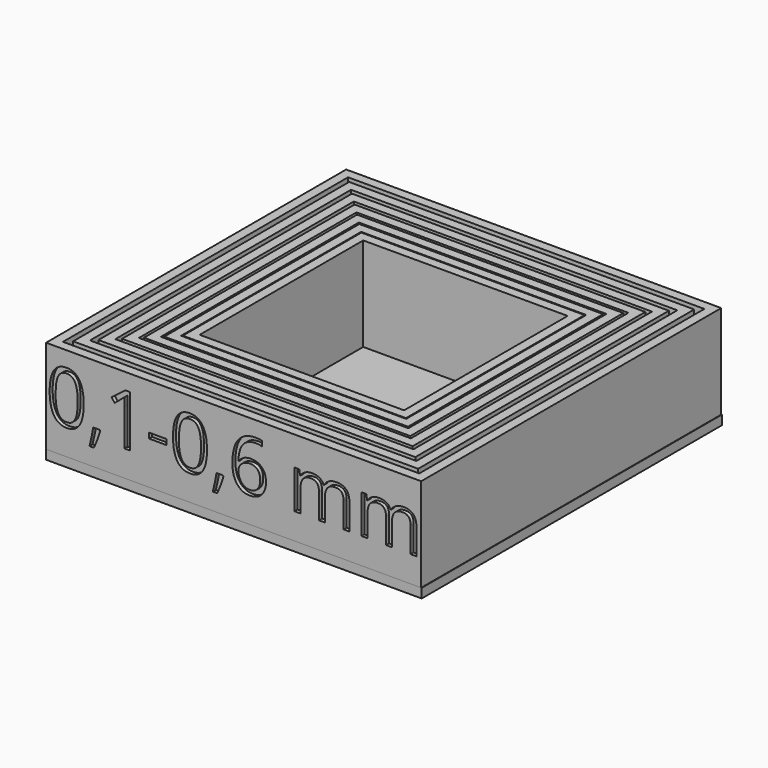
from build123d import *

# Parameters (mm, degrees)
F1_W         = 40.056457743
F1_H         = 40.0194465183
F2_DEPTH     = 1
F0_W         = 40
F0_H         = 40
F0_W_2       = 38
F0_H_2       = 38
F0_W_3       = 36.8
F0_H_3       = 36.8
F0_W_4       = 34.8
F0_H_4       = 34.8
F0_W_5       = 33.8
F0_H_5       = 33.8
F0_W_6       = 31.8
F0_H_6       = 31.8
F0_W_7       = 31
F0_H_7       = 31
F0_W_8       = 29
F0_H_8       = 29
F0_W_9       = 28.4
F0_H_9       = 28.4
F0_W_10      = 26.4
F0_H_10      = 26.4
F0_W_11      = 26
F0_H_11      = 26
F0_W_12      = 24
F0_H_12      = 24
F0_W_13      = 23.8
F0_H_13      = 23.8
F0_W_14      = 21.8
F0_H_14      = 21.8
F3_DEPTH     = 10
F4_TEXT_SIZE = 7.6881494384
F5_DEPTH     = 0.4


# Not quite as in the source:
# - Text() gives the source's letters only with a copy of the font that has no kerning and outlines rounded to 1/6400 em; it was checked with that copy


with BuildPart() as f2:
    # F1 (on Top) → F2 (new body)
    with BuildSketch(Plane.XY):
        with Locations((24.7721569613, -17.6345624495)):
            Rectangle(F1_W, F1_H)
    extrude(amount=-F2_DEPTH)

    # F0 (on Top) → F3 (join)
    with BuildSketch(Plane.XY):
        with Locations((24.7547212243, -17.6580692828)):
            Rectangle(F0_W, F0_H)
        with Locations((24.7547212243, -17.6580692828)):
            Rectangle(F0_W_2, F0_H_2, mode=Mode.SUBTRACT)
        with Locations((24.7547212243, -17.6580692828)):
            Rectangle(F0_W_3, F0_H_3)
        with Locations((24.7547212243, -17.6580692828)):
            Rectangle(F0_W_4, F0_H_4, mode=Mode.SUBTRACT)
        with Locations((24.7547212243, -17.6580692828)):
            Rectangle(F0_W_5, F0_H_5)
        with Locations((24.7547212243, -17.6580692828)):
            Rectangle(F0_W_6, F0_H_6, mode=Mode.SUBTRACT)
        with Locations((24.7547212243, -17.6580692828)):
            Rectangle(F0_W_7, F0_H_7)
        with Locations((24.7547212243, -17.6580692828)):
            Rectangle(F0_W_8, F0_H_8, mode=Mode.SUBTRACT)
        with Locations((24.7547212243, -17.6580692828)):
            Rectangle(F0_W_9, F0_H_9)
        with Locations((24.7547212243, -17.6580692828)):
            Rectangle(F0_W_10, F0_H_10, mode=Mode.SUBTRACT)
        with Locations((24.7547212243, -17.6580692828)):
            Rectangle(F0_W_11, F0_H_11)
        with Locations((24.7547212243, -17.6580692828)):
            Rectangle(F0_W_12, F0_H_12, mode=Mode.SUBTRACT)
        with Locations((24.7547212243, -17.6580692828)):
            Rectangle(F0_W_13, F0_H_13)
        with Locations((24.7547212243, -17.6580692828)):
            Rectangle(F0_W_14, F0_H_14, mode=Mode.SUBTRACT)
    extrude(amount=F3_DEPTH)

    # F4 (on face) → F5 (cut)
    with BuildSketch(Plane.XZ.offset(37.6580692828)):
        with Locations((4.7547212243, 2.7874156917)):
            Text('0,1-0,6 mm', F4_TEXT_SIZE, font='Open Sans', text_align=(TextAlign.LEFT, TextAlign.BOTTOM))
    extrude(amount=-F5_DEPTH, mode=Mode.SUBTRACT)


solid = f2.part
